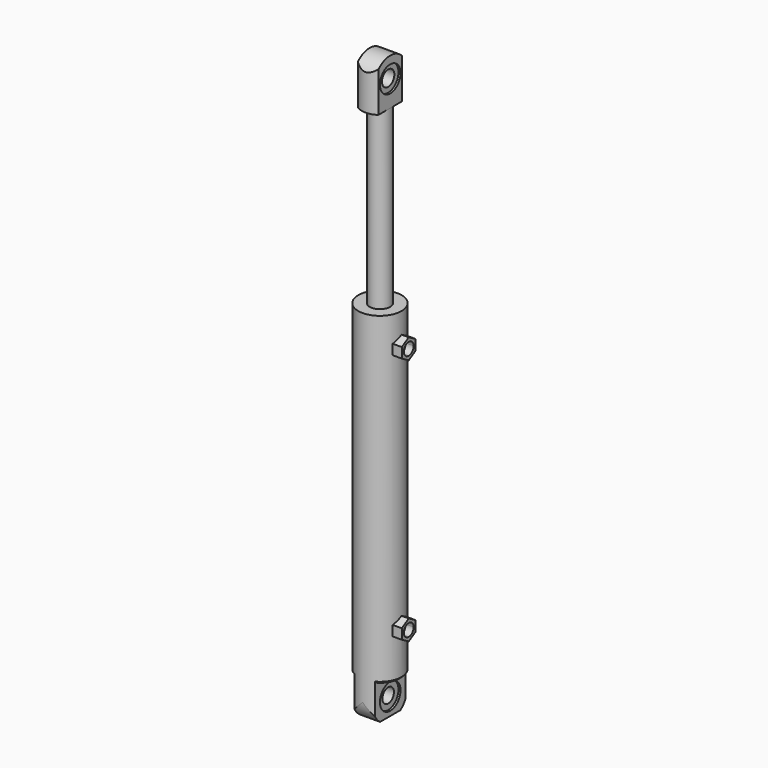
from build123d import *

# Parameters (mm, degrees)
F0_R      = 21
F1_DEPTH  = 315
F2_R      = 10
F3_DEPTH  = 300
F4_R      = 21
F5_DEPTH  = 35
F6_W      = 15.6832183711
F6_H      = 49.8256795108
F6_W_2    = 16.2493828684
F6_H_2    = 44.8511093855
F7_DEPTH  = 35
F8_R      = 12.5
F9_DEPTH  = 2
F10_R     = 7
F11_DEPTH = 25
F12_R     = 12.5
F13_DEPTH = 2
F15_DEPTH = 25
F16_SIZE  = 2
F17_R     = 10
F18_DEPTH = 200
F19_R     = 10
F20_DEPTH = 50
F21_R     = 17.5
F21_R_2   = 10
F22_DEPTH = 30
F23_R     = 17.5
F24_DEPTH = 20
F26_DEPTH = 60
F28_DEPTH = 2
F29_R     = 7.5
F30_DEPTH = 25
F31_R     = 12.5
F31_R_2   = 7.5
F32_DEPTH = 2
F34_DEPTH = 25
F36_DEPTH = 18


with BuildPart() as f1:
    # F0 (on Top) → F1 (new body)
    with BuildSketch(Plane.XY):
        Circle(F0_R)
    extrude(amount=F1_DEPTH)

    # F2 (on face) → F3 (cut)
    with BuildSketch(Plane.XY.offset(315)):
        Circle(F2_R)
    extrude(amount=-F3_DEPTH, mode=Mode.SUBTRACT)

    # F4 (on face) → F5 (join)
    with BuildSketch(Plane.XY):
        Circle(F4_R)
    extrude(amount=-F5_DEPTH)

    # F6 (on face) → F7 (cut)
    with BuildSketch(Plane(origin=(0, 0, -35), x_dir=(1, 0, 0), z_dir=(0, 0, -1))):
        with Locations((17.8416091856, -0.4472155124)):
            Rectangle(F6_W, F6_H)
        with Locations((-18.1246914342, 1.4644041657)):
            Rectangle(F6_W_2, F6_H_2)
    extrude(amount=-F7_DEPTH, mode=Mode.SUBTRACT)

    # F8 (on face) → F9 (cut)
    with BuildSketch(Plane(origin=(-10, 0, 0), x_dir=(0, -1, 0), z_dir=(-1, 0, 0))):
        with Locations((0, -18)):
            Circle(F8_R)
    extrude(amount=-F9_DEPTH, mode=Mode.SUBTRACT)

    # F10 (on face) → F11 (cut)
    with BuildSketch(Plane(origin=(-8, 0, 0), x_dir=(0, -1, 0), z_dir=(-1, 0, 0))):
        with Locations((0, -18)):
            Circle(F10_R)
    extrude(amount=-F11_DEPTH, mode=Mode.SUBTRACT)

    # F12 (on face) → F13 (cut)
    with BuildSketch(Plane.YZ.offset(10)):
        with Locations((0, -18)):
            Circle(F12_R)
    extrude(amount=-F13_DEPTH, mode=Mode.SUBTRACT)

    # F14 (on face) → F15 (cut)
    with BuildSketch(Plane(origin=(-10, 0, 0), x_dir=(0, -1, 0), z_dir=(-1, 0, 0))):
        with BuildLine():
            ThreePointArc((21, -18), (0, -39), (-21, -18))
            Line((-21, -18), (-30, -18))
            ThreePointArc((-30, -18), (0, -48), (30, -18))
            Line((30, -18), (21, -18))
        make_face()
    extrude(amount=-F15_DEPTH, mode=Mode.SUBTRACT)

    # F16
    f16_edges = [f1.edges().sort_by_distance(p)[0] for p in [
        (18.041619, 10.747093, 0),
        (18.041619, -10.747093, 0),
        (-21, 0, 0),
    ]]
    chamfer(f16_edges, length=F16_SIZE)

    # F35 (on face) → F36 (join)
    with BuildSketch(Plane.YZ.offset(10)):
        with BuildLine():
            Line((0, 50.508012673), (0, 54.3229672492))
            Line((0, 54.3229672492), (-8.5, 49.4154899611))
            Line((-8.5, 49.4154899611), (-8.5, 39.6005353849))
            Line((-8.5, 39.6005353849), (0, 34.6930580967))
            Line((0, 34.6930580967), (0, 38.508012673))
            ThreePointArc((0, 38.508012673), (-6, 44.508012673), (0, 50.508012673))
        make_face()
        with BuildLine():
            Line((-8.5, 280.0925227119), (0, 275.1850454238))
            Line((0, 275.1850454238), (0, 279))
            ThreePointArc((0, 279), (-6, 285), (0, 291))
            Line((0, 291), (0, 294.8149545762))
            Line((0, 294.8149545762), (-8.5, 289.9074772881))
            Line((-8.5, 289.9074772881), (-8.5, 280.0925227119))
        make_face()
        with BuildLine():
            Line((0, 279), (0, 275.1850454238))
            Line((0, 275.1850454238), (8.5, 280.0925227119))
            Line((8.5, 280.0925227119), (8.5, 289.9074772881))
            Line((8.5, 289.9074772881), (0, 294.8149545762))
            Line((0, 294.8149545762), (0, 291))
            ThreePointArc((0, 291), (4.2426406871, 289.2426406871), (6, 285))
            ThreePointArc((6, 285), (4.2426406871, 280.7573593129), (0, 279))
        make_face()
        with BuildLine():
            Line((8.5, 49.4154899611), (0, 54.3229672492))
            Line((0, 54.3229672492), (0, 50.508012673))
            ThreePointArc((0, 50.508012673), (4.2426406871, 48.7506533601), (6, 44.508012673))
            ThreePointArc((6, 44.508012673), (4.2426406871, 40.2653719858), (0, 38.508012673))
            Line((0, 38.508012673), (0, 34.6930580967))
            Line((0, 34.6930580967), (0.1884949477, 34.8018857055))
            Line((0.1884949477, 34.8018857055), (8.5, 39.6005353849))
            Line((8.5, 39.6005353849), (8.5, 49.4154899611))
        make_face()
    extrude(amount=F36_DEPTH)


with BuildPart() as f18:
    # F17 (on face) → F18 (new body)
    with BuildSketch(Plane.XY.offset(315)):
        Circle(F17_R)
    extrude(amount=F18_DEPTH)

    # F19 (on face) → F20 (join)
    with BuildSketch(Plane(origin=(0, 0, 315), x_dir=(1, 0, 0), z_dir=(0, 0, -1))):
        Circle(F19_R)
    extrude(amount=F20_DEPTH)

    # F21 (on face) → F22 (join)
    with BuildSketch(Plane.XY.offset(515)):
        Circle(F21_R)
        Circle(F21_R_2, mode=Mode.SUBTRACT)
        Circle(F21_R_2)
    extrude(amount=-F22_DEPTH)

    # F23 (on face) → F24 (join)
    with BuildSketch(Plane.XY.offset(515)):
        Circle(F23_R)
    extrude(amount=F24_DEPTH)

    # F25 (on face) → F26 (cut)
    with BuildSketch(Plane.XY.offset(535)):
        with BuildLine():
            ThreePointArc((-10, 14.3614066163), (-17.5, 0), (-10, -14.3614066163))
            Line((-10, -14.3614066163), (-10, 14.3614066163))
        make_face()
        with BuildLine():
            ThreePointArc((17.5, 0), (15.5120920575, 8.100925873), (10, 14.3614066163))
            Line((10, 14.3614066163), (10, -14.3614066163))
            ThreePointArc((10, -14.3614066163), (15.5120920575, -8.100925873), (17.5, 0))
        make_face()
    extrude(amount=-F26_DEPTH, mode=Mode.SUBTRACT)

    # F27 (on face) → F28 (cut)
    with BuildSketch(Plane(origin=(-10, 0, 0), x_dir=(0, -1, 0), z_dir=(-1, 0, 0))):
        with BuildLine():
            ThreePointArc((12.5, 510), (8.8388347648, 518.8388347648), (0, 522.5))
            Line((0, 522.5), (0, 497.5))
            ThreePointArc((0, 497.5), (8.8388347648, 501.1611652352), (12.5, 510))
        make_face()
        with BuildLine():
            Line((0, 497.5), (0, 522.5))
            ThreePointArc((0, 522.5), (-12.5, 510), (0, 497.5))
        make_face()
    extrude(amount=-F28_DEPTH, mode=Mode.SUBTRACT)

    # F29 (on face) → F30 (cut)
    with BuildSketch(Plane(origin=(-8, 0, 0), x_dir=(0, -1, 0), z_dir=(-1, 0, 0))):
        with Locations((0, 510)):
            Circle(F29_R)
    extrude(amount=-F30_DEPTH, mode=Mode.SUBTRACT)

    # F31 (on face) → F32 (cut)
    with BuildSketch(Plane.YZ.offset(10)):
        with Locations((0, 510)):
            Circle(F31_R)
        with Locations((0, 510)):
            Circle(F31_R_2, mode=Mode.SUBTRACT)
        with Locations((0, 510)):
            Circle(F31_R)
    extrude(amount=-F32_DEPTH, mode=Mode.SUBTRACT)

    # F33 (on face) → F34 (cut)
    with BuildSketch(Plane(origin=(-10, 0, 0), x_dir=(0, -1, 0), z_dir=(-1, 0, 0))):
        with BuildLine():
            ThreePointArc((-20, 510), (0, 530), (20, 510))
            Line((20, 510), (33.9818404813, 510))
            ThreePointArc((33.9818404813, 510), (0, 543.9818404813), (-33.9818404813, 510))
            Line((-33.9818404813, 510), (-20, 510))
        make_face()
    extrude(amount=-F34_DEPTH, mode=Mode.SUBTRACT)


solid = Compound([f1.part, f18.part])
